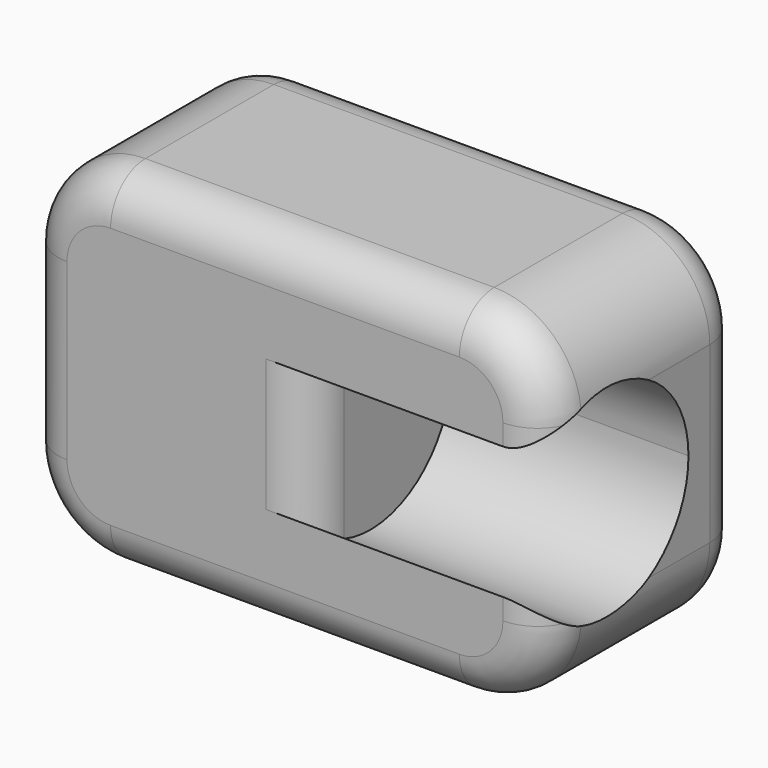
from build123d import *

# Parameters (mm, degrees)
F0_W         = 152.4
F0_H         = 101.6
F1_DEPTH     = 72.136
F3_DEPTH     = 69.088
F4_T1_DEPTH  = 199.136
F5_T1_DEPTH  = 101.6
F5_T3_DEPTH  = 50.8
F5_T5_DEPTH  = 37.8518945456
F5_T7_DEPTH  = 37.8518945456
F5_T12_DEPTH = 102.0962109088
F5_S13_R     = 29.4462721735
F5_T14_DEPTH = 53
F5_T16_ANGLE = 89.9999999994
F5_T18_ANGLE = 89.9999999994
F5_T20_ANGLE = 89.9999999994
F5_T22_ANGLE = 89.9999999994
F5_T24_ANGLE = 89.9999999994
F5_T26_ANGLE = 89.9999999994
F5_T28_ANGLE = 89.9999999994
F5_T30_ANGLE = 89.9999999994


# Not quite as in the source:
# - a fillet or chamfer that OpenCascade refuses, or shapes differently, is made with other operations: its cross-section is extruded or revolved along the edge and cut away or added


with BuildPart() as f1:
    # F0 (on Front) → F1 (new body)
    with BuildSketch(Plane.XZ):
        Rectangle(F0_W, F0_H)
    extrude(amount=F1_DEPTH)

    # F2 (on face) → F3 (cut)
    with BuildSketch(Plane.YZ.offset(76.2)):
        with BuildLine():
            Line((-72.136, -19.2981054544), (-72.136, 19.2981054544))
            ThreePointArc((-72.136, 19.2981054544), (-79.3411824793, 0), (-72.136, -19.2981054544))
        make_face()
        with BuildLine():
            ThreePointArc((-72.136, -19.2981054544), (-39.5952558372, -27.5862295855), (-20.4486381322, 0))
            ThreePointArc((-20.4486381322, 0), (-39.5952558372, 27.5862295855), (-72.136, 19.2981054544))
            Line((-72.136, 19.2981054544), (-72.136, -19.2981054544))
        make_face()
    extrude(amount=-F3_DEPTH, mode=Mode.SUBTRACT)

    # F4: fillet of radius 25.4 on 4 edges, made by hand

    # F4_s2 → F4_t1 (cut)
    with BuildSketch(Plane.XZ.offset(-63.5)):
        with BuildLine():
            ThreePointArc((50.8, -50.8), (68.7605122421, -43.3605122421), (76.2, -25.4))
            Line((76.2, -25.4), (76.2, -50.8))
            Line((76.2, -50.8), (50.8, -50.8))
        make_face()
        with BuildLine():
            ThreePointArc((-50.8, -50.8), (-68.7605122421, -43.3605122421), (-76.2, -25.4))
            Line((-76.2, -25.4), (-76.2, -50.8))
            Line((-76.2, -50.8), (-50.8, -50.8))
        make_face()
        with BuildLine():
            ThreePointArc((76.2, 25.4), (68.7605122421, 43.3605122421), (50.8, 50.8))
            Line((50.8, 50.8), (76.2, 50.8))
            Line((76.2, 50.8), (76.2, 25.4))
        make_face()
        with BuildLine():
            ThreePointArc((-76.2, 25.4), (-68.7605122421, 43.3605122421), (-50.8, 50.8))
            Line((-50.8, 50.8), (-76.2, 50.8))
            Line((-76.2, 50.8), (-76.2, 25.4))
        make_face()
    extrude(amount=F4_T1_DEPTH, mode=Mode.SUBTRACT)

    # F5: fillet of radius 12.7 on 16 edges, made by hand

    # F5_s2 → F5_t1 (cut)
    with BuildSketch(Plane.YZ.offset(-50.8)):
        with BuildLine():
            ThreePointArc((-72.136, 38.1), (-68.4162561211, 47.0802561211), (-59.436, 50.8))
            Line((-59.436, 50.8), (-72.136, 50.8))
            Line((-72.136, 50.8), (-72.136, 38.1))
        make_face()
        with BuildLine():
            ThreePointArc((0, 38.1), (-3.7197438789, 47.0802561211), (-12.7, 50.8))
            Line((-12.7, 50.8), (0, 50.8))
            Line((0, 50.8), (0, 38.1))
        make_face()
        with BuildLine():
            ThreePointArc((-12.7, -50.8), (-3.7197438789, -47.0802561211), (0, -38.1))
            Line((0, -38.1), (0, -50.8))
            Line((0, -50.8), (-12.7, -50.8))
        make_face()
        with BuildLine():
            ThreePointArc((-59.436, -50.8), (-68.4162561211, -47.0802561211), (-72.136, -38.1))
            Line((-72.136, -38.1), (-72.136, -50.8))
            Line((-72.136, -50.8), (-59.436, -50.8))
        make_face()
    extrude(amount=F5_T1_DEPTH, mode=Mode.SUBTRACT)

    # F5_s4 → F5_t3 (cut)
    with BuildSketch(Plane.XY.offset(-25.4)):
        with BuildLine():
            ThreePointArc((-63.5, 0), (-72.4802561211, -3.7197438789), (-76.2, -12.7))
            Line((-76.2, -12.7), (-76.2, 0))
            Line((-76.2, 0), (-63.5, 0))
        make_face()
        with BuildLine():
            ThreePointArc((63.5, 0), (72.4802561211, -3.7197438789), (76.2, -12.7))
            Line((76.2, -12.7), (76.2, 0))
            Line((76.2, 0), (63.5, 0))
        make_face()
        with BuildLine():
            ThreePointArc((-63.5, -72.136), (-72.4802561211, -68.4162561211), (-76.2, -59.436))
            Line((-76.2, -59.436), (-76.2, -72.136))
            Line((-76.2, -72.136), (-63.5, -72.136))
        make_face()
    extrude(amount=F5_T3_DEPTH, mode=Mode.SUBTRACT)

    # F5_s6 → F5_t5 (cut)
    with BuildSketch(Plane.XY.offset(-12.4518945456)):
        with BuildLine():
            ThreePointArc((63.5, -72.136), (72.4802561211, -68.4162561211), (76.2, -59.436))
            Line((76.2, -59.436), (76.2, -72.136))
            Line((76.2, -72.136), (63.5, -72.136))
        make_face()
    extrude(amount=F5_T5_DEPTH, mode=Mode.SUBTRACT)

    # F5_s8 → F5_t7 (cut)
    with BuildSketch(Plane.XY.offset(-25.4)):
        with BuildLine():
            ThreePointArc((63.5, -72.136), (72.4802561211, -68.4162561211), (76.2, -59.436))
            Line((76.2, -59.436), (76.2, -72.136))
            Line((76.2, -72.136), (63.5, -72.136))
        make_face()
    extrude(amount=F5_T7_DEPTH, mode=Mode.SUBTRACT)


with BuildPart() as f5_tool10:
    # F5_s11 → F5_t12 (new body)
    with BuildSketch(Plane.XY.offset(-51.0481054544)):
        with BuildLine():
            ThreePointArc((-5.588, -72.136), (3.3922561211, -68.4162561211), (7.112, -59.436))
            Line((7.112, -59.436), (7.112, -72.136))
            Line((7.112, -72.136), (-5.588, -72.136))
        make_face()
    extrude(amount=F5_T12_DEPTH)

    # F5_s13 → F5_t14 (intersect, symmetric)
    with BuildSketch(Plane.YZ.offset(0.8)):
        with Locations((-49.8949103057, 0)):
            Circle(F5_S13_R)
    extrude(amount=F5_T14_DEPTH, both=True, mode=Mode.INTERSECT)


with BuildPart() as f1_1:
    add(f1.part)

    # F5_t9: cut F5_tool10
    add(f5_tool10.part, mode=Mode.SUBTRACT)

    # F5_s15 → F5_t16 (revolve, cut)
    with BuildSketch(Plane.YZ.offset(-50.7999999999)):
        with BuildLine():
            ThreePointArc((0, -38.1), (-3.7197438789, -47.0802561211), (-12.7, -50.8))
            Line((-12.7, -50.8), (0, -50.8))
            Line((0, -50.8), (0, -38.1))
        make_face()
    revolve(axis=Axis((-50.7999999999, 0, -25.3999999999), (0, 1, 0)), revolution_arc=F5_T16_ANGLE, mode=Mode.SUBTRACT)

    # F5_s17 → F5_t18 (revolve, cut)
    with BuildSketch(Plane.XY.offset(25.3999999999)):
        with BuildLine():
            ThreePointArc((-63.5, 0), (-72.4802561211, -3.7197438789), (-76.2, -12.7))
            Line((-76.2, -12.7), (-76.2, 0))
            Line((-76.2, 0), (-63.5, 0))
        make_face()
    revolve(axis=Axis((-50.7999999999, 0, 25.3999999999), (0, 1, 0)), revolution_arc=F5_T18_ANGLE, mode=Mode.SUBTRACT)

    # F5_s19 → F5_t20 (revolve, cut)
    with BuildSketch(Plane.YZ.offset(50.7999999999)):
        with BuildLine():
            ThreePointArc((0, 38.1), (-3.7197438789, 47.0802561211), (-12.7, 50.8))
            Line((-12.7, 50.8), (0, 50.8))
            Line((0, 50.8), (0, 38.1))
        make_face()
    revolve(axis=Axis((50.7999999999, 0, 25.3999999999), (0, 1, 0)), revolution_arc=F5_T20_ANGLE, mode=Mode.SUBTRACT)

    # F5_s21 → F5_t22 (revolve, cut)
    with BuildSketch(Plane.XY.offset(-25.3999999999)):
        with BuildLine():
            ThreePointArc((63.5, 0), (72.4802561211, -3.7197438789), (76.2, -12.7))
            Line((76.2, -12.7), (76.2, 0))
            Line((76.2, 0), (63.5, 0))
        make_face()
    revolve(axis=Axis((50.7999999999, 0, -25.3999999999), (0, 1, 0)), revolution_arc=F5_T22_ANGLE, mode=Mode.SUBTRACT)

    # F5_s23 → F5_t24 (revolve, cut)
    with BuildSketch(Plane.XY.offset(-25.3999999999)):
        with BuildLine():
            ThreePointArc((76.2, -59.436), (72.4802561211, -68.4162561211), (63.5, -72.136))
            Line((63.5, -72.136), (76.2, -72.136))
            Line((76.2, -72.136), (76.2, -59.436))
        make_face()
    revolve(axis=Axis((50.7999999999, -72.136, -25.3999999999), (0, 1, 0)), revolution_arc=F5_T24_ANGLE, mode=Mode.SUBTRACT)

    # F5_s25 → F5_t26 (revolve, cut)
    with BuildSketch(Plane.XY.offset(25.3999999999)):
        with BuildLine():
            ThreePointArc((-63.5, -72.136), (-72.4802561211, -68.4162561211), (-76.2, -59.436))
            Line((-76.2, -59.436), (-76.2, -72.136))
            Line((-76.2, -72.136), (-63.5, -72.136))
        make_face()
    revolve(axis=Axis((-50.7999999999, -72.136, 25.3999999999), (0, 1, 0)), revolution_arc=F5_T26_ANGLE, mode=Mode.SUBTRACT)

    # F5_s27 → F5_t28 (revolve, cut)
    with BuildSketch(Plane.YZ.offset(50.7999999999)):
        with BuildLine():
            ThreePointArc((-72.136, 38.1), (-68.4162561211, 47.0802561211), (-59.436, 50.8))
            Line((-59.436, 50.8), (-72.136, 50.8))
            Line((-72.136, 50.8), (-72.136, 38.1))
        make_face()
    revolve(axis=Axis((50.7999999999, -72.136, 25.3999999999), (0, 1, 0)), revolution_arc=F5_T28_ANGLE, mode=Mode.SUBTRACT)

    # F5_s29 → F5_t30 (revolve, cut)
    with BuildSketch(Plane.YZ.offset(-50.7999999999)):
        with BuildLine():
            ThreePointArc((-72.136, -38.1), (-68.4162561211, -47.0802561211), (-59.436, -50.8))
            Line((-59.436, -50.8), (-72.136, -50.8))
            Line((-72.136, -50.8), (-72.136, -38.1))
        make_face()
    revolve(axis=Axis((-50.7999999999, -72.136, -25.3999999999), (0, 1, 0)), revolution_arc=F5_T30_ANGLE, mode=Mode.SUBTRACT)


solid = f1_1.part
